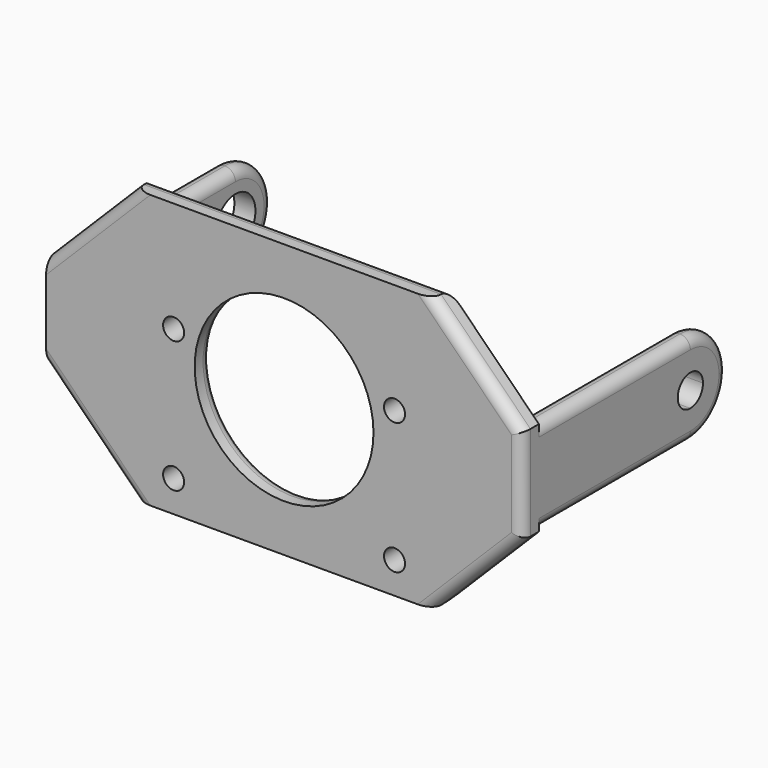
from build123d import *

# Parameters (mm, degrees)
F0_W     = 45.25
F0_H     = 26
F0_W_2   = 25
F0_H_2   = 24
F0_R     = 1
F0_R_2   = 8.5
F1_DEPTH = 2
F3_DEPTH = 2
F4_R     = 1
F5_DEPTH = 2
F6_SIZE  = 8.5
F7_R     = 1
F7_R_2   = 0.99999


# Not quite as in the source:
# - a fillet or chamfer is up to 0.001 mm smaller than in the source, because OpenCascade refuses the exact size


with BuildPart() as f1:
    # F0 (on Front) → F1 (new body)
    with BuildSketch(Plane.XZ):
        Rectangle(F0_W, F0_H)
        Rectangle(F0_W_2, F0_H_2, mode=Mode.SUBTRACT)
        Rectangle(F0_W_2, F0_H_2)
        with Locations((-10.5, -10)):
            Circle(F0_R, mode=Mode.SUBTRACT)
        with Locations((10.5, -10)):
            Circle(F0_R, mode=Mode.SUBTRACT)
        with Locations((-10.5, 2.5)):
            Circle(F0_R, mode=Mode.SUBTRACT)
        Circle(F0_R_2, mode=Mode.SUBTRACT)
        with Locations((10.5, 2.5)):
            Circle(F0_R, mode=Mode.SUBTRACT)
    extrude(amount=-F1_DEPTH)

    # F2 (on face) → F3 (join)
    with BuildSketch(Plane.YZ.offset(22.625)):
        with BuildLine():
            ThreePointArc((20, -4.4), (15.6, 0), (20, 4.4))
            Line((20, 4.4), (2, 4.4))
            Line((2, 4.4), (2, -4.4))
            Line((2, -4.4), (20, -4.4))
        make_face()
        with BuildLine():
            ThreePointArc((20, 1.5), (21.0606601718, 1.0606601718), (21.5, 0))
            ThreePointArc((21.5, 0), (21.0606601718, -1.0606601718), (20, -1.5))
            Line((20, -1.5), (20, -4.4))
            ThreePointArc((20, -4.4), (23.1112698372, -3.1112698372), (24.4, 0))
            ThreePointArc((24.4, 0), (23.1112698372, 3.1112698372), (20, 4.4))
            Line((20, 4.4), (20, 1.5))
        make_face()
        with BuildLine():
            ThreePointArc((20, -1.5), (18.5, 0), (20, 1.5))
            Line((20, 1.5), (20, 4.4))
            ThreePointArc((20, 4.4), (15.6, 0), (20, -4.4))
            Line((20, -4.4), (20, -1.5))
        make_face()
    extrude(amount=-F3_DEPTH)

    # F4 (on face) → F5 (join)
    with BuildSketch(Plane(origin=(-22.625, 0, 0), x_dir=(0, -1, 0), z_dir=(-1, 0, 0))):
        with BuildLine():
            ThreePointArc((-20, -2.375), (-22.375, 0), (-20, 2.375))
            Line((-20, 2.375), (-20, 4.4))
            ThreePointArc((-20, 4.4), (-24.4, 0), (-20, -4.4))
            Line((-20, -4.4), (-20, -2.375))
        make_face()
        with BuildLine():
            ThreePointArc((-20, 2.375), (-18.3206213947, 1.6793786053), (-17.625, 0))
            ThreePointArc((-17.625, 0), (-18.3206213947, -1.6793786053), (-20, -2.375))
            Line((-20, -2.375), (-20, -4.4))
            ThreePointArc((-20, -4.4), (-16.8887301628, -3.1112698372), (-15.6, 0))
            ThreePointArc((-15.6, 0), (-16.8887301628, 3.1112698372), (-20, 4.4))
            Line((-20, 4.4), (-20, 2.375))
        make_face()
        with BuildLine():
            Line((-2, 4.4), (-20, 4.4))
            ThreePointArc((-20, 4.4), (-16.8887301628, 3.1112698372), (-15.6, 0))
            ThreePointArc((-15.6, 0), (-16.8887301628, -3.1112698372), (-20, -4.4))
            Line((-20, -4.4), (-2, -4.4))
            Line((-2, -4.4), (-2, 4.4))
        make_face()
        with Locations((-13.33, 0)):
            Circle(F4_R, mode=Mode.SUBTRACT)
        with Locations((-7.33, 0)):
            Circle(F4_R, mode=Mode.SUBTRACT)
    extrude(amount=-F5_DEPTH)

    # F6
    f6_edges = [f1.edges().sort_by_distance(p)[0] for p in [
        (22.625, 1, 13),
        (-22.625, 1, 13),
        (-22.625, 1, -13),
        (22.625, 1, -13),
    ]]
    chamfer(f6_edges, length=F6_SIZE)

    # F7 (call 1 of 10: OpenCascade refuses the feature's edges together)
    f7_edges = [f1.edges().sort_by_distance(p)[0] for p in [
        (-8.5, 2, 0),
    ]]
    fillet(f7_edges, radius=F7_R)

    # F7#2 (call 2 of 10)
    f7_2_edges = [f1.edges().sort_by_distance(p)[0] for p in [
        (18.375, 0, 8.75),
        (18.375, 0, -8.75),
        (22.625, 0, 0),
    ]]
    fillet(f7_2_edges, radius=F7_R)

    # F7#3 (call 3 of 10)
    f7_3_edges = [f1.edges().sort_by_distance(p)[0] for p in [
        (-18.375, 0, -8.75),
    ]]
    fillet(f7_3_edges, radius=F7_R)

    # F7#4 (call 4 of 10)
    f7_4_edges = [f1.edges().sort_by_distance(p)[0] for p in [
        (-18.375, 0, 8.75),
    ]]
    fillet(f7_4_edges, radius=F7_R)

    # F7#5 (call 5 of 10)
    f7_5_edges = [f1.edges().sort_by_distance(p)[0] for p in [
        (-22.625, 11, -4.4),
    ]]
    fillet(f7_5_edges, radius=F7_R)

    # F7#6 (call 6 of 10)
    f7_6_edges = [f1.edges().sort_by_distance(p)[0] for p in [
        (22.625, 11, 4.4),
    ]]
    fillet(f7_6_edges, radius=F7_R)

    # F7#7 (call 7 of 10)
    f7_7_edges = [f1.edges().sort_by_distance(p)[0] for p in [
        (0, 2, -13),
    ]]
    fillet(f7_7_edges, radius=F7_R)

    # F7#8 (call 8 of 10)
    f7_8_edges = [f1.edges().sort_by_distance(p)[0] for p in [
        (0, 2, 13),
    ]]
    fillet(f7_8_edges, radius=F7_R)

    # F7#9 (call 9 of 10) (radius 1 in the source; OpenCascade refuses exactly that, so slightly less here)
    f7_9_edges = [f1.edges().sort_by_distance(p)[0] for p in [
        (-20.625, 11, 4.4),
    ]]
    fillet(f7_9_edges, radius=F7_R_2)

    # F7#10 (call 10 of 10) (radius 1 in the source; OpenCascade refuses exactly that, so slightly less here)
    f7_10_edges = [f1.edges().sort_by_distance(p)[0] for p in [
        (20.625, 11, 4.4),
    ]]
    fillet(f7_10_edges, radius=F7_R_2)


solid = f1.part
